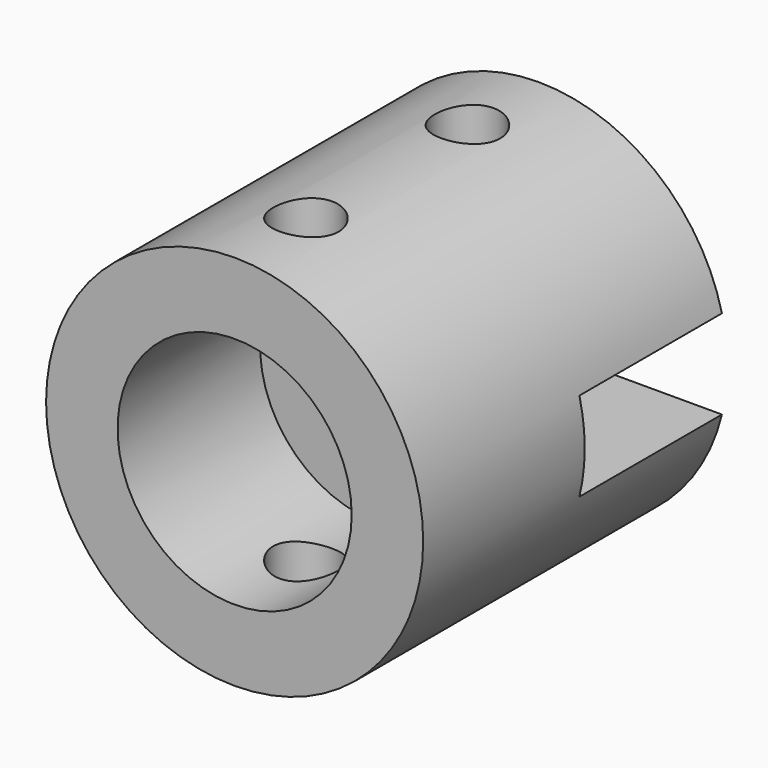
from build123d import *

# Parameters (mm, degrees)
F0_R     = 31.75
F1_DEPTH = 64
F2_R     = 19.7125485486
F3_DEPTH = 30
F5_DEPTH = 30
F6_R     = 5.5
F7_DEPTH = 35
F8_R     = 5.5
F9_DEPTH = 35


# Not quite as in the source:
# - the program builds the solid bodies; features that only make, move or delete a surface that nothing else refers to are left out


with BuildPart() as f1:
    # F0 (on Front) → F1 (new body)
    with BuildSketch(Plane.XZ):
        Circle(F0_R)
    extrude(amount=F1_DEPTH)

    # F2 (on face) → F3 (cut)
    with BuildSketch(Plane.XZ.offset(64)):
        Circle(F2_R)
    extrude(amount=-F3_DEPTH, mode=Mode.SUBTRACT)

    # F4 (on face) → F5 (cut)
    with BuildSketch(Plane(origin=(0, 0, 0), x_dir=(-1, 0, 0), z_dir=(0, 1, 0))):
        with BuildLine():
            Line((-30.8514586365, -7.5), (30.8514586365, -7.5))
            ThreePointArc((30.8514586365, -7.5), (31.5245643246, -3.7768166682), (31.75, 0))
            ThreePointArc((31.75, 0), (31.5245643246, 3.7768166682), (30.8514586365, 7.5))
            Line((30.8514586365, 7.5), (-30.8514586365, 7.5))
            ThreePointArc((-30.8514586365, 7.5), (-31.75, 0), (-30.8514586365, -7.5))
        make_face()
    extrude(amount=-F5_DEPTH, mode=Mode.SUBTRACT)

    # F6 (on Top) → F7 (cut, symmetric)
    with BuildSketch(Plane.XY):
        with Locations((0, -49)):
            Circle(F6_R)
    extrude(amount=F7_DEPTH, both=True, mode=Mode.SUBTRACT)

    # F8 (on Top) → F9 (cut, symmetric)
    with BuildSketch(Plane.XY):
        with Locations((0, -15)):
            Circle(F8_R)
    extrude(amount=F9_DEPTH, both=True, mode=Mode.SUBTRACT)


solid = f1.part
